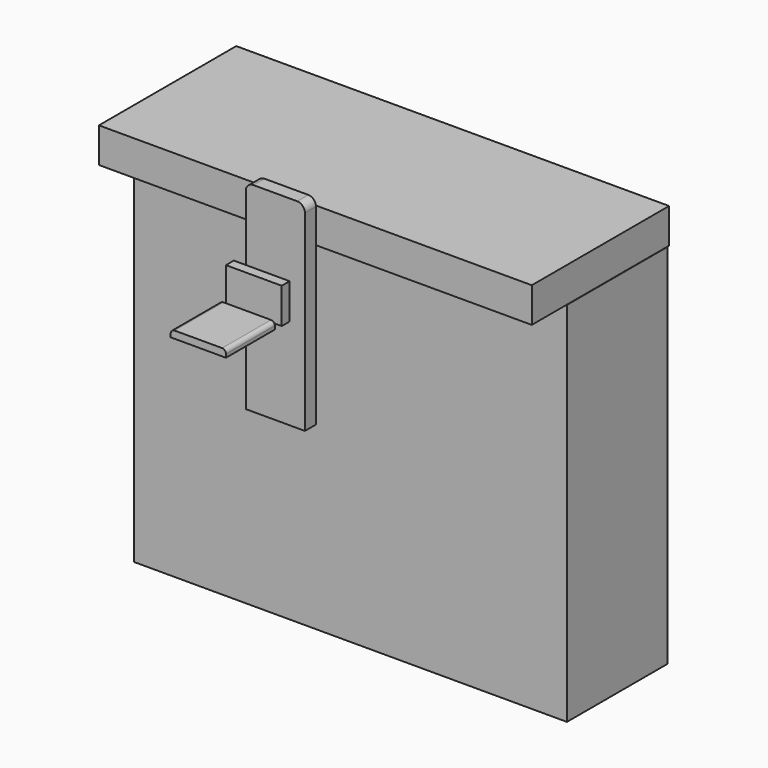
from build123d import *

# Parameters (mm, degrees)
F0_W         = 38.795568049
F0_H         = 131.0027092695
F1_DEPTH     = 9.0788379312
F2_W         = 36.6244800389
F2_H         = 6.4905062318
F3_DEPTH     = 23.3007315546
F4_W         = 36.2693443894
F4_H         = 40.0586724281
F5_DEPTH     = 4.7574751079
F6_R         = 2.54
F7_W         = 112.597361207
F7_H         = 22.9164585471
F9_DEPTH     = 159.4235897064
F8_W         = 82.463145256
F8_H         = 127.2133886814
F10_DEPTH    = 124.53237921
F12_DEPTH    = 113.6232465506
F13_T1_DEPTH = 21.7788379312


# Not quite as in the source:
# - a fillet or chamfer that OpenCascade refuses, or shapes differently, is made with other operations: its cross-section is extruded or revolved along the edge and cut away or added


with BuildPart() as f1:
    # F0 (on Front) → F1 (new body)
    with BuildSketch(Plane.XZ):
        with Locations((-1.533780247, -1.2631490827)):
            Rectangle(F0_W, F0_H)
    extrude(amount=F1_DEPTH)

    # F7 (on Right) → F9 (join)
    with BuildSketch(Plane.YZ):
        with Locations((56.2986806035, 48.2688806951)):
            Rectangle(F7_W, F7_H)
    extrude(amount=F9_DEPTH)

    # F10#2 (add): a face of the model
    f10_2_faces = [f1.faces().sort_by_distance(p)[0] for p in [
        (0, 56.2986806035, 48.2688806951),
    ]]
    extrude(f10_2_faces, amount=F10_DEPTH)


with BuildPart() as f3:
    # F2 (on Top) → F3 (new body)
    with BuildSketch(Plane.XY):
        with Locations((-2.2713560611, -22.5855186582)):
            Rectangle(F2_W, F2_H)
    extrude(amount=F3_DEPTH)


with BuildPart() as f5:
    # F4 (on Top) → F5 (new body)
    with BuildSketch(Plane.XY):
        with Locations((-2.4360008538, -51.0658025742)):
            Rectangle(F4_W, F4_H)
    extrude(amount=F5_DEPTH)

    # F6
    f6_edges = [f5.edges().sort_by_distance(p)[0] for p in [
        (15.698671, -51.065803, 4.757475),
        (-20.570673, -51.065803, 4.757475),
    ]]
    fillet(f6_edges, radius=F6_R)


with BuildPart() as f9:
    # F8 (on Right) → F9, piece 2 (new body)
    with BuildSketch(Plane.YZ):
        with Locations((70.1026767492, -26.9764810801)):
            Rectangle(F8_W, F8_H)
    extrude(amount=F9_DEPTH)

    # F10 (add): a face of the model
    f10_faces = [f9.faces().sort_by_distance(p)[0] for p in [
        (0, 70.1026767492, -26.9764810801),
    ]]
    extrude(f10_faces, amount=F10_DEPTH)

    # F11: union F1
    add(f1.part)

    # F12 (add): a face of the model
    f12_faces = [f9.faces().sort_by_distance(p)[0] for p in [
        (17.4456052482, 70.1026767492, -90.5831754208),
    ]]
    extrude(f12_faces, amount=F12_DEPTH)

    # F13: fillet of radius 5.08 on 2 edges, made by hand

    # F13_s2 → F13_t1 (cut)
    with BuildSketch(Plane.XZ):
        with BuildLine():
            ThreePointArc((12.7840037775, 64.2382055521), (16.3761062259, 62.7503080005), (17.8640037775, 59.1582055521))
            Line((17.8640037775, 59.1582055521), (17.8640037775, 64.2382055521))
            Line((17.8640037775, 64.2382055521), (12.7840037775, 64.2382055521))
        make_face()
        with BuildLine():
            ThreePointArc((-15.8515642715, 64.2382055521), (-19.4436667199, 62.7503080005), (-20.9315642715, 59.1582055521))
            Line((-20.9315642715, 59.1582055521), (-20.9315642715, 64.2382055521))
            Line((-20.9315642715, 64.2382055521), (-15.8515642715, 64.2382055521))
        make_face()
    extrude(amount=F13_T1_DEPTH, mode=Mode.SUBTRACT)


solid = Compound([f3.part, f5.part, f9.part])
